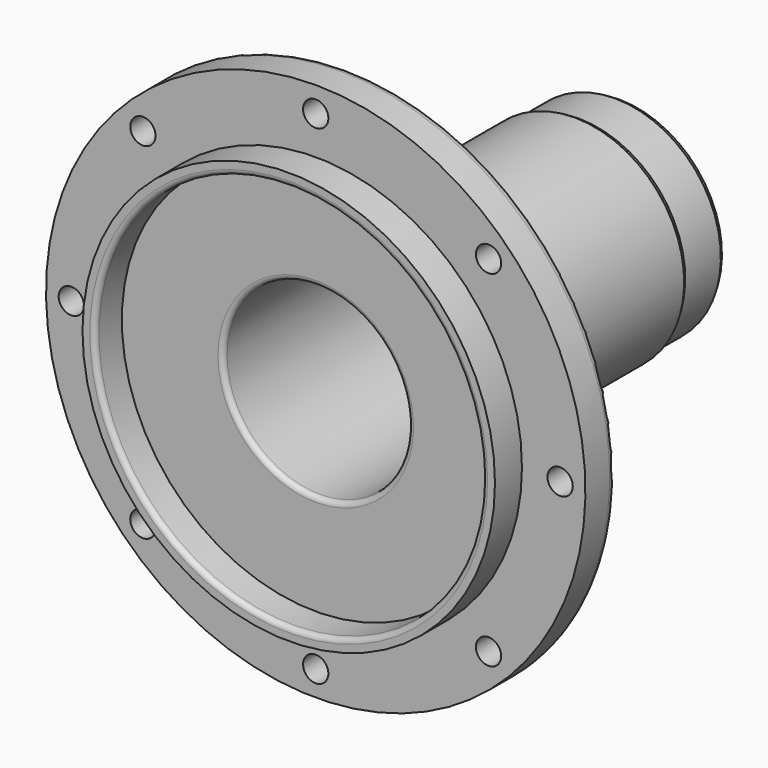
from build123d import *

# Parameters (mm, degrees)
F2_R            = 4.7625
F3_DEPTH        = 25.4
F3_COPIES_COUNT = 8
F4_R            = 34.925
F5_DEPTH        = 152.4
F7_SIZE2        = 1.0998522628
F7_SIZE         = 1.905
F8_R            = 3.175
F9_R            = 77.6986
F9_R_2          = 73.025
F10_DEPTH       = 12.7
F11_R           = 1.905


# Not quite as in the source:
# - a fillet or chamfer that OpenCascade refuses, or shapes differently, is made with other operations: its cross-section is extruded or revolved along the edge and cut away or added
# - a pattern or mirror of a feature is missing from the dataset's text; its kind, count and spacing are read off the source's solid


with BuildPart() as f1:
    # F0 (on Right) → F1 (revolve)
    with BuildSketch(Plane.YZ):
        Polygon((-150.5628967822, 101.6), (-165.1678967822, 101.6), (-165.1678967822, 0), (-22.2928967822, 0), (-22.2928967822, 39.8399), (-41.3428967822, 39.8399), (-41.3428967822, 41.25595), (-123.8928967822, 41.25595), (-123.8928967822, 47.6504), (-150.5628967822, 47.6504), align=None)
    revolve(axis=Axis((0, -0.5433106927, 0), (0, 1, 0)))

    # F2 (on face) → F3 (cut)
    with BuildSketch(Plane(origin=(0, -150.5628967822, 0), x_dir=(-1, 0, 0), z_dir=(0, 1, 0))):
        with Locations((0, 92.075)):
            Circle(F2_R)
    f3 = extrude(amount=-F3_DEPTH, mode=Mode.SUBTRACT)

    # F3_copies: F3 ×8 about axis
    f3_copies_axis = Axis((0, 0, 0), (0, 1, 0))
    for i in range(1, F3_COPIES_COUNT):
        add(f3.rotate(f3_copies_axis, i * 360 / F3_COPIES_COUNT), mode=Mode.SUBTRACT)

    # F4 (on face) → F5 (cut)
    with BuildSketch(Plane(origin=(0, -22.2928967822, 0), x_dir=(-1, 0, 0), z_dir=(0, 1, 0))):
        Circle(F4_R)
    extrude(amount=-F5_DEPTH, mode=Mode.SUBTRACT)

    # F6: chamfer of 1.905 x 1.0998522628 on 1 edges, made by hand

    # F6_s1 → F6_t2 (revolve, cut)
    with BuildSketch(Plane.YZ):
        Polygon((-22.2928967822, 38.7400477372), (-24.1978967822, 39.8399), (-22.2928967822, 39.8399), align=None)
    revolve(axis=Axis((0, -22.2928967822, 0), (0, 1, 0)), mode=Mode.SUBTRACT)

    # F7
    f7_edges = [f1.edges().sort_by_distance(p)[0] for p in [
        (0, -41.342897, -41.25595),
    ]]
    chamfer(f7_edges, length=F7_SIZE, length2=F7_SIZE2)

    # F8
    f8_edges = [f1.edges().sort_by_distance(p)[0] for p in [
        (0, -123.892897, -41.25595),
        (0, -150.562897, -47.6504),
        (0, -150.562897, -101.6),
    ]]
    fillet(f8_edges, radius=F8_R)

    # F9 (on face) → F10 (join)
    with BuildSketch(Plane.XZ.offset(165.1678967822)):
        Circle(F9_R)
        Circle(F9_R_2, mode=Mode.SUBTRACT)
    extrude(amount=F10_DEPTH)

    # F11
    f11_edges = [f1.edges().sort_by_distance(p)[0] for p in [
        (-73.025, -177.867897, 0),
        (34.925, -165.167897, 0),
    ]]
    fillet(f11_edges, radius=F11_R)


solid = f1.part
